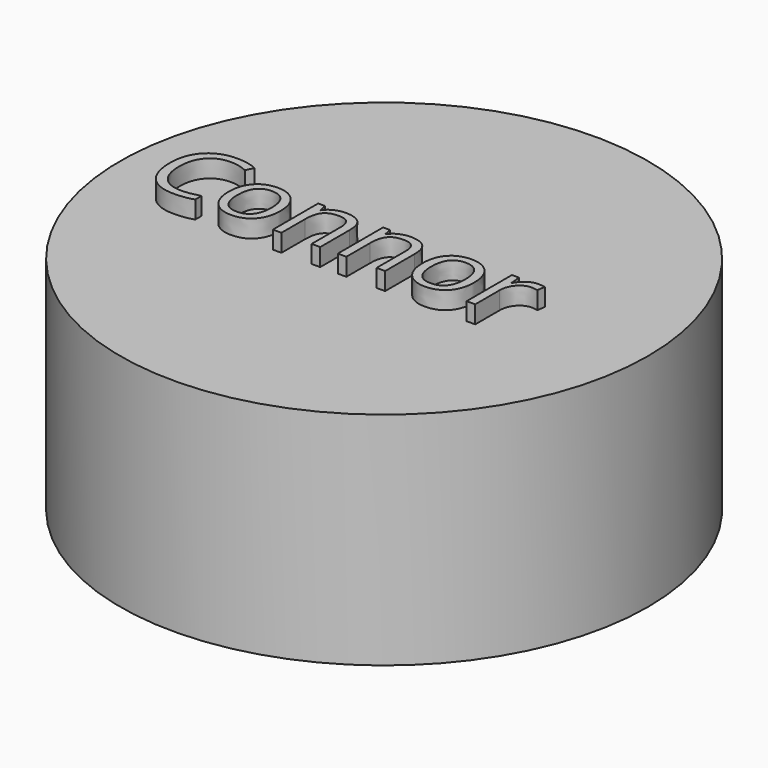
from build123d import *

# Parameters (mm, degrees)
F0_R         = 29.8849307276
F1_DEPTH     = 25
F2_TEXT_SIZE = 11.9768545523
F3_DEPTH     = 2


# Not quite as in the source:
# - the program builds the solid bodies; features that only make, move or delete a surface that nothing else refers to are left out
# - Text() gives the source's letters only with a copy of the font that has no kerning and outlines rounded to 1/6400 em; it was checked with that copy


with BuildPart() as f1:
    # F0 (on Top) → F1 (new body)
    with BuildSketch(Plane.XY):
        Circle(F0_R)
    extrude(amount=F1_DEPTH)

    # F2 (on face) → F3 (join)
    with BuildSketch(Plane.XY.offset(25)):
        with Locations((-24.5639290661, -4.8123626038)):
            Text('Connor', F2_TEXT_SIZE, font='Open Sans', text_align=(TextAlign.LEFT, TextAlign.BOTTOM))
    extrude(amount=F3_DEPTH)


solid = f1.part
